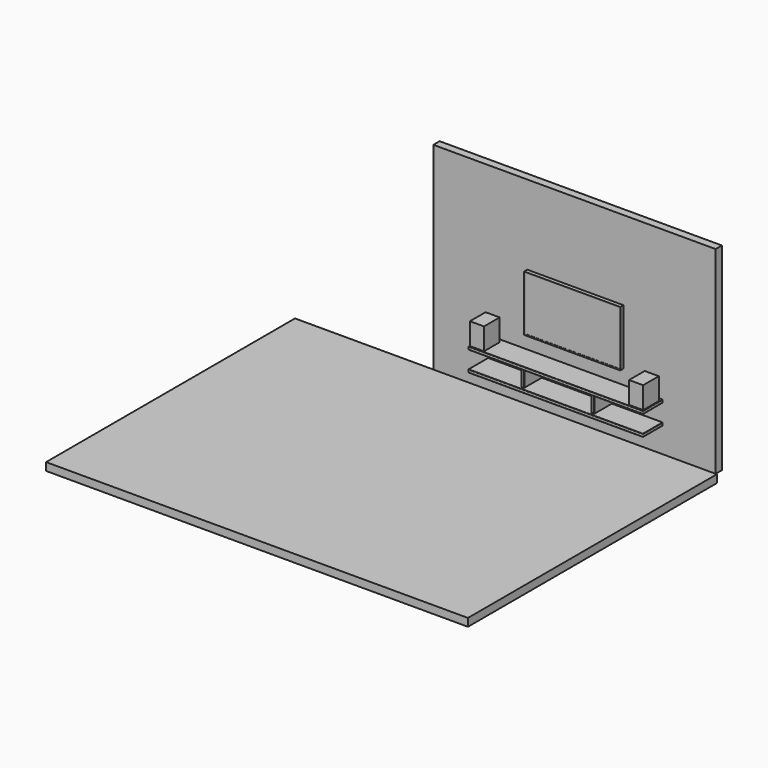
from build123d import *

# Parameters (mm, degrees)
F0_W      = 3610
F0_H      = 2530
F1_DEPTH  = 100
F2_W      = 5394.8676586151
F2_H      = 3978.9967536926
F3_DEPTH  = 100
F4_W      = 1230
F4_H      = 715
F5_DEPTH  = 50
F6_W      = 1210
F6_H      = 690
F7_DEPTH  = 2
F8_W      = 2235
F8_H      = 38
F9_DEPTH  = 315
F10_W     = 38
F10_H     = 220
F11_DEPTH = 280
F12_R     = 5
F12_2_R   = 5
F13_R     = 5
F13_2_R   = 5
F14_W     = 180
F14_H     = 250
F15_DEPTH = 280


with BuildPart() as f1:
    # F0 (on Front) → F1 (new body)
    with BuildSketch(Plane.XZ):
        with Locations((0, 1265)):
            Rectangle(F0_W, F0_H)
    extrude(amount=-F1_DEPTH)


with BuildPart() as f3:
    # F2 (on Top) → F3 (new body)
    with BuildSketch(Plane.XY):
        with Locations((-877.255320549, -1989.4983768463)):
            Rectangle(F2_W, F2_H)
    extrude(amount=-F3_DEPTH)


with BuildPart() as f5:
    # F4 (on face) → F5 (new body)
    with BuildSketch(Plane.XZ):
        with Locations((10, 1157.5)):
            Rectangle(F4_W, F4_H)
    extrude(amount=F5_DEPTH)

    # F6 (on face) → F7 (cut)
    with BuildSketch(Plane.XZ.offset(50)):
        with Locations((10, 1160)):
            Rectangle(F6_W, F6_H)
    extrude(amount=-F7_DEPTH, mode=Mode.SUBTRACT)


with BuildPart() as f9:
    # F8 (on face) → F9 (new body)
    with BuildSketch(Plane.XZ):
        with Locations((10, 597)):
            Rectangle(F8_W, F8_H)
    extrude(amount=F9_DEPTH)

    # F12
    f12_edges = [f9.edges().sort_by_distance(p)[0] for p in [
        (-1107.5, -315, 597),
        (-1107.5, -157.5, 616),
        (-1107.5, -157.5, 578),
        (10, -315, 578),
        (10, -315, 616),
        (1127.5, -157.5, 616),
        (1127.5, -157.5, 578),
        (1127.5, -315, 597),
    ]]
    fillet(f12_edges, radius=F12_R)


with BuildPart() as f9b:
    # F8 (on face) → F9, piece 2 (new body)
    with BuildSketch(Plane.XZ):
        with Locations((10, 339)):
            Rectangle(F8_W, F8_H)
    extrude(amount=F9_DEPTH)

    # F12#2
    f12_2_edges = [f9b.edges().sort_by_distance(p)[0] for p in [
        (-1107.5, -157.5, 358),
        (-1107.5, -157.5, 320),
        (-1107.5, -315, 339),
        (10, -315, 320),
        (1127.5, -315, 339),
        (1127.5, -157.5, 320),
        (1127.5, -157.5, 358),
        (10, -315, 358),
    ]]
    fillet(f12_2_edges, radius=F12_2_R)


with BuildPart() as f11:
    # F10 (on face) → F11 (new body)
    with BuildSketch(Plane.XZ):
        with Locations((-438.5, 468)):
            Rectangle(F10_W, F10_H)
    extrude(amount=F11_DEPTH)

    # F13
    f13_edges = [f11.edges().sort_by_distance(p)[0] for p in [
        (-457.5, -280, 468),
        (-419.5, -280, 468),
    ]]
    fillet(f13_edges, radius=F13_R)


with BuildPart() as f11b:
    # F10 (on face) → F11, piece 2 (new body)
    with BuildSketch(Plane.XZ):
        with Locations((458.5, 468)):
            Rectangle(F10_W, F10_H)
    extrude(amount=F11_DEPTH)

    # F13#2
    f13_2_edges = [f11b.edges().sort_by_distance(p)[0] for p in [
        (439.5, -280, 468),
        (477.5, -280, 468),
    ]]
    fillet(f13_2_edges, radius=F13_2_R)


with BuildPart() as f15:
    # F14 (on face) → F15 (new body)
    with BuildSketch(Plane.XY.offset(616)):
        with Locations((-1007.5, -175)):
            Rectangle(F14_W, F14_H)
    extrude(amount=F15_DEPTH)


with BuildPart() as f15b:
    # F14 (on face) → F15, piece 2 (new body)
    with BuildSketch(Plane.XY.offset(616)):
        with Locations((1027.5, -175)):
            Rectangle(F14_W, F14_H)
    extrude(amount=F15_DEPTH)


solid = Compound([f1.part, f3.part, f5.part, f9.part, f9b.part, f11.part, f11b.part, f15.part, f15b.part])
